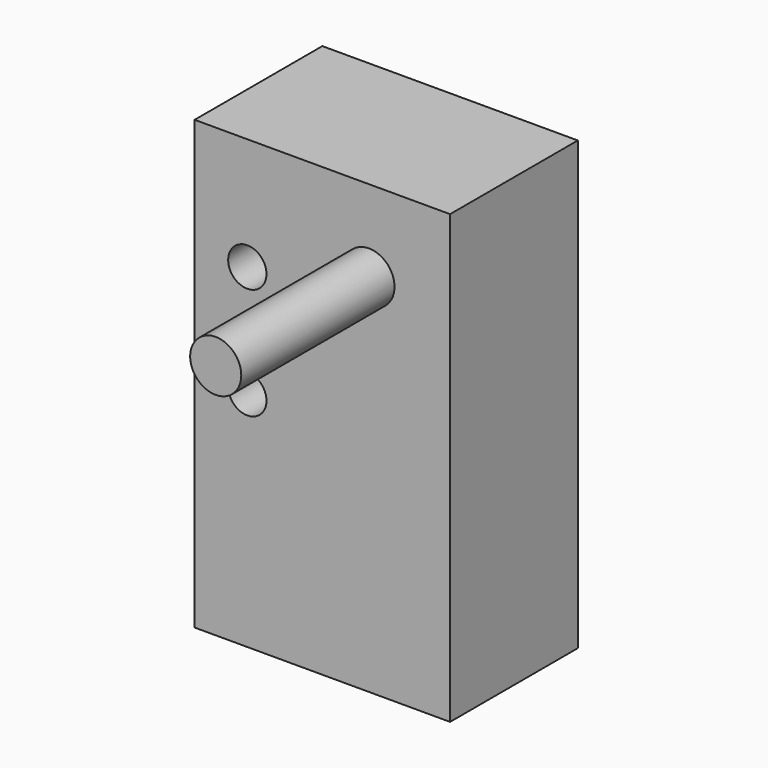
from build123d import *

# Parameters (mm, degrees)
F0_W     = 40
F0_H     = 70
F1_DEPTH = 25
F2_R     = 4
F3_DEPTH = 30
F6_D     = 6


# Not quite as in the source:
# - the program builds the solid bodies; features that only make, move or delete a surface that nothing else refers to are left out


with BuildPart() as f1:
    # F0 (on Front) → F1 (new body)
    with BuildSketch(Plane.XZ):
        with Locations((20, 35)):
            Rectangle(F0_W, F0_H)
    extrude(amount=F1_DEPTH)

    # F2 (on face) → F3 (join)
    with BuildSketch(Plane.XZ.offset(25)):
        with Locations((27.3, 57.15)):
            Circle(F2_R)
    extrude(amount=F3_DEPTH)

    # F6 (through all)
    with Locations(Plane(origin=(0, 0, 0), x_dir=(1, 0, 0), z_dir=(0, 1, 0))):
        with Locations((8.25, -52.3875), (8.25, -34.925)):
            Hole(F6_D / 2)


solid = f1.part
